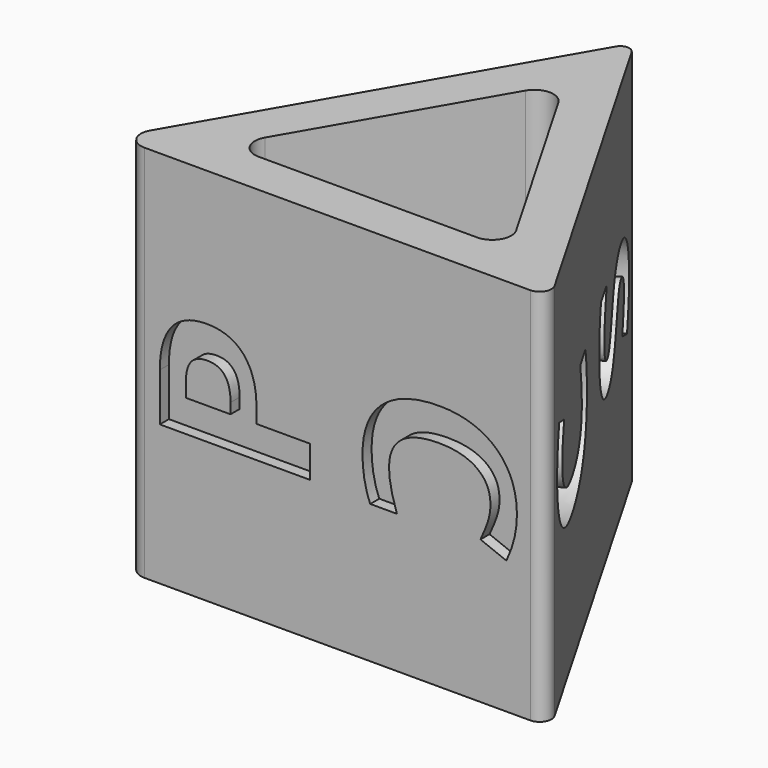
from build123d import *

# Parameters (mm, degrees)
F1_DEPTH     = 20
F2_TEXT_SIZE = 11.1111111111
F5_DEPTH     = 1
F3_TEXT_SIZE = 11.1111111111
F6_DEPTH     = 0.6
F4_TEXT_SIZE = 11.1111111111
F7_DEPTH     = 0.6


# Not quite as in the source:
# - Text() gives the source's letters only with a copy of the font that has no kerning and outlines rounded to 1/6400 em; it was checked with that copy


with BuildPart() as f1:
    # F0 (on Top) → F1 (new body)
    with BuildSketch(Plane.XY):
        with BuildLine():
            Line((-9.9554491924, -6.6395280957), (10.4241991924, -6.6395280957))
            ThreePointArc((10.4241991924, -6.6395280957), (10.9620995962, -6.3289711528), (10.9620995962, -5.7078572669))
            Line((10.9620995962, -5.7078572669), (0.4114799492, 12.566352013))
            ThreePointArc((0.4114799492, 12.566352013), (0, 12.8039200724), (-0.4114799492, 12.566352013))
            Line((-0.4114799492, 12.566352013), (-10.7277245962, -5.3019078589))
            ThreePointArc((-10.7277245962, -5.3019078589), (-10.7277245962, -6.1936546834), (-9.9554491924, -6.6395280957))
        make_face()
        with BuildLine():
            ThreePointArc((6.6339745962, -2.8301270189), (6.6339745962, -3.8301270189), (5.7679491924, -4.3301270189))
            Line((5.7679491924, -4.3301270189), (-5.7679491924, -4.3301270189))
            ThreePointArc((-5.7679491924, -4.3301270189), (-6.6339745962, -3.8301270189), (-6.6339745962, -2.8301270189))
            Line((-6.6339745962, -2.8301270189), (-0.8660254038, 7.1602540378))
            ThreePointArc((-0.8660254038, 7.1602540378), (0, 7.6602540378), (0.8660254038, 7.1602540378))
            Line((0.8660254038, 7.1602540378), (6.6339745962, -2.8301270189))
        make_face(mode=Mode.SUBTRACT)
    extrude(amount=F1_DEPTH)

    # F2 (on face) → F5 (cut)
    with BuildSketch(Plane(origin=(5.75, 3.3197640478, 0), x_dir=(-0.5, 0.8660254038, 0), z_dir=(0.8660254038, 0.5, 0))):
        with Locations(Location((-1.6741991924, 6.2951388889), (0, 0, 90))):
            Text('C', F2_TEXT_SIZE, font='Open Sans', font_style=FontStyle.BOLD, text_align=(TextAlign.LEFT, TextAlign.BOTTOM))
        with Locations(Location((1.9270401015, 13.2005208333), (0, 0, -90))):
            Text('S', F2_TEXT_SIZE, font='Open Sans', font_style=FontStyle.BOLD, text_align=(TextAlign.LEFT, TextAlign.BOTTOM))
    extrude(amount=-F5_DEPTH, mode=Mode.SUBTRACT)

    # F3 (on face) → F6 (cut)
    with BuildSketch(Plane(origin=(-5.75, 3.3197640478, 0), x_dir=(-0.5, -0.8660254038, 0), z_dir=(-0.8660254038, 0.5, 0))):
        with Locations(Location((-1.9270401015, 6.7994791667), (0, 0, 90))):
            Text('S', F3_TEXT_SIZE, font='Open Sans', font_style=FontStyle.BOLD, text_align=(TextAlign.LEFT, TextAlign.BOTTOM))
        with Locations(Location((1.2054491924, 13.5989583333), (0, 0, -90))):
            Text('P', F3_TEXT_SIZE, font='Open Sans', font_style=FontStyle.BOLD, text_align=(TextAlign.LEFT, TextAlign.BOTTOM))
    extrude(amount=-F6_DEPTH, mode=Mode.SUBTRACT)

    # F4 (on face) → F7 (cut)
    with BuildSketch(Plane.XZ.offset(6.6395280957)):
        with Locations(Location((-1.2054491924, 6.4010416667), (0, 0, 90))):
            Text('P', F4_TEXT_SIZE, font='Open Sans', font_style=FontStyle.BOLD, text_align=(TextAlign.LEFT, TextAlign.BOTTOM))
        with Locations(Location((1.6741991924, 13.7048611111), (0, 0, -90))):
            Text('C', F4_TEXT_SIZE, font='Open Sans', font_style=FontStyle.BOLD, text_align=(TextAlign.LEFT, TextAlign.BOTTOM))
    extrude(amount=-F7_DEPTH, mode=Mode.SUBTRACT)


solid = f1.part
